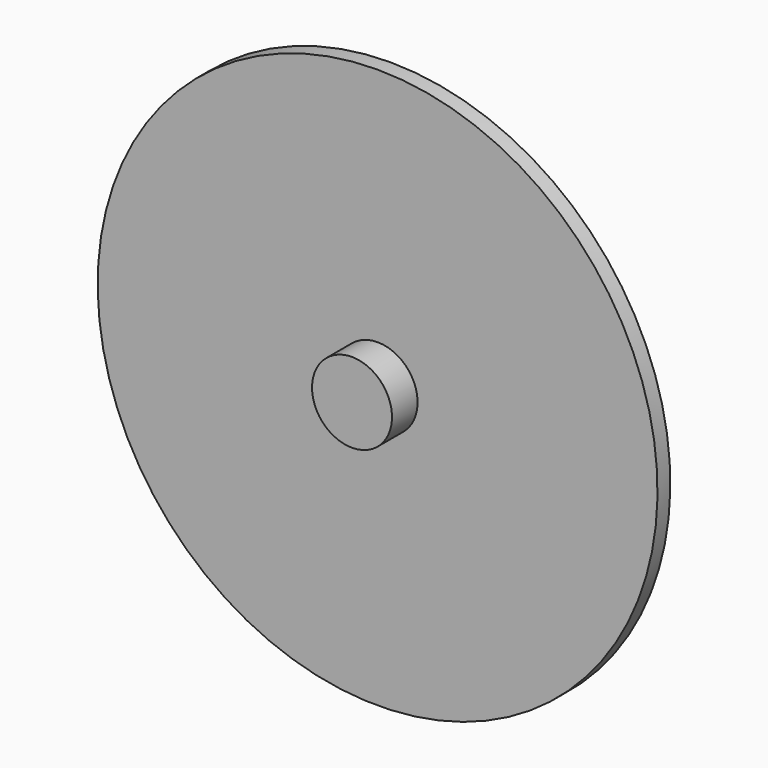
from build123d import *

# Parameters (mm, degrees)
F0_W     = 1
F0_H     = 17.5
F2_R     = 2.5
F3_DEPTH = 3
F4_DEPTH = 6


with BuildPart() as f1:
    # F0 (on Right) → F1 (revolve)
    with BuildSketch(Plane.YZ):
        with Locations((-0.5, 8.75)):
            Rectangle(F0_W, F0_H)
    revolve(axis=Axis((0, -0.5, 0), (0, 1, 0)))

    # F2 (on face) → F3 (join)
    with BuildSketch(Plane(origin=(0, 0, 0), x_dir=(-1, 0, 0), z_dir=(0, 1, 0))):
        Circle(F2_R)
    extrude(amount=F3_DEPTH)

    # F4 (add): a face of the model
    f4_faces = [f1.faces().sort_by_distance(p)[0] for p in [
        (0, 3, 0),
    ]]
    extrude(f4_faces, amount=-F4_DEPTH)


solid = f1.part
